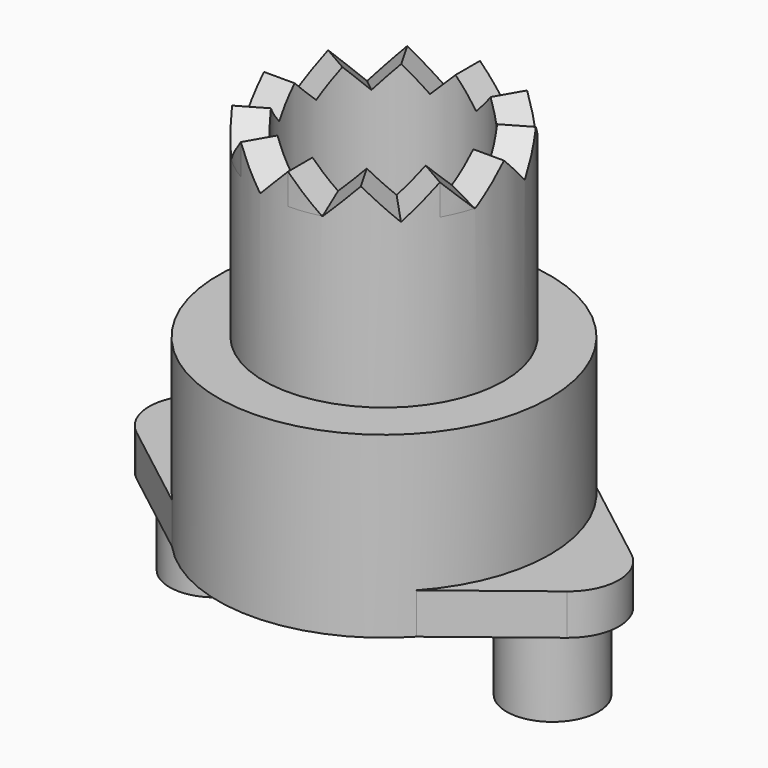
from build123d import *

# Parameters (mm, degrees)
F0_R          = 8.75
F1_DEPTH      = 2
F2_R          = 16.25
F3_DEPTH      = 17.5
F4_R          = 11.75
F5_DEPTH      = 19
F6_R          = 8.75
F7_DEPTH      = 33
F8_R          = 4
F9_DEPTH      = 5.5
F11_DEPTH     = 4
F12_R         = 4.5
F13_DEPTH     = 8
F15_DEPTH     = 22
F17_DEPTH     = 3
F18_SIZE      = 2.99999
F19_SIZE      = 2.99999
F20_DEPTH     = 3
F21_SIZE      = 2.99999
F22_T4_DEPTH  = 18.4300979278
F22_S5_R      = 11.75
F22_T6_DEPTH  = 11
F22_S7_R      = 8.75
F22_T8_DEPTH  = 11
F22_T13_DEPTH = 18.4300979278
F22_S14_R     = 11.75
F22_T15_DEPTH = 12
F22_S17_R     = 8.75
F22_T18_DEPTH = 12
F22_T22_DEPTH = 18.4300979278
F22_S23_R     = 11.75
F22_T24_DEPTH = 12
F22_S25_R     = 8.75
F22_T26_DEPTH = 12
F23_SIZE      = 2.99999
F24_SIZE      = 2.99999
F25_DEPTH     = 3
F26_T4_DEPTH  = 18.4300979278
F26_S5_R      = 11.75
F26_T6_DEPTH  = 12
F26_S7_R      = 8.75
F26_T8_DEPTH  = 12
F26_T12_DEPTH = 18.4300979278
F26_S13_R     = 11.75
F26_T14_DEPTH = 12
F26_S15_R     = 8.75
F26_T16_DEPTH = 12
F26_T20_DEPTH = 18.4300979278
F26_S21_R     = 11.75
F26_T22_DEPTH = 12
F26_S23_R     = 8.75
F26_T24_DEPTH = 12
F26_T28_DEPTH = 18.4300979278
F26_S29_R     = 11.75
F26_T30_DEPTH = 11
F26_S31_R     = 8.75
F26_T32_DEPTH = 11
F26_T36_DEPTH = 18.4300979278
F26_S37_R     = 11.75
F26_T38_DEPTH = 11
F26_S39_R     = 8.75
F26_T40_DEPTH = 11
F26_T44_DEPTH = 18.4300979278
F26_S45_R     = 11.75
F26_T46_DEPTH = 12
F26_S47_R     = 8.75
F26_T48_DEPTH = 12
F26_T52_DEPTH = 18.4300979278
F26_S53_R     = 11.75
F26_T54_DEPTH = 12
F26_S55_R     = 8.75
F26_T56_DEPTH = 12
F26_T60_DEPTH = 18.4300979278
F26_S61_R     = 11.75
F26_T62_DEPTH = 11
F26_S63_R     = 8.75
F26_T64_DEPTH = 11
F26_T68_DEPTH = 18.4300979278
F26_S69_R     = 11.75
F26_T70_DEPTH = 12
F26_S71_R     = 8.75
F26_T72_DEPTH = 12
F26_T76_DEPTH = 18.4300979278
F26_S77_R     = 11.75
F26_T78_DEPTH = 11
F26_S79_R     = 8.75
F26_T80_DEPTH = 11
F26_T84_DEPTH = 18.4300979278
F26_S85_R     = 11.75
F26_T86_DEPTH = 12
F26_S87_R     = 8.75
F26_T88_DEPTH = 12
F26_T92_DEPTH = 18.4300979278
F26_S93_R     = 11.75
F26_T94_DEPTH = 12
F26_S95_R     = 8.75
F26_T96_DEPTH = 12


# Not quite as in the source:
# - a fillet or chamfer that OpenCascade refuses, or shapes differently, is made with other operations: its cross-section is extruded or revolved along the edge and cut away or added
# - a fillet or chamfer is up to 0.001 mm smaller than in the source, because OpenCascade refuses the exact size


with BuildPart() as f1:
    # F0 (on Top) → F1 (new body)
    with BuildSketch(Plane.XY):
        Circle(F0_R)
    extrude(amount=F1_DEPTH)

    # F2 (on face) → F3 (join)
    with BuildSketch(Plane.XY.offset(2)):
        Circle(F2_R)
    extrude(amount=F3_DEPTH)

    # F4 (on face) → F5 (join)
    with BuildSketch(Plane.XY.offset(19.5)):
        Circle(F4_R)
    extrude(amount=F5_DEPTH)

    # F6 (on face) → F7 (cut)
    with BuildSketch(Plane.XY.offset(38.5)):
        Circle(F6_R)
    extrude(amount=-F7_DEPTH, mode=Mode.SUBTRACT)

    # F8 (on face) → F9 (cut, through all)
    with BuildSketch(Plane(origin=(0, 0, 0), x_dir=(1, 0, 0), z_dir=(0, 0, -1))):
        Circle(F8_R)
    extrude(amount=-F9_DEPTH, mode=Mode.SUBTRACT)

    # F10 (on face) → F11 (join)
    with BuildSketch(Plane(origin=(0, 0, 2), x_dir=(1, 0, 0), z_dir=(0, 0, -1))):
        with BuildLine():
            ThreePointArc((-11.9608737139, -11), (-16.25, 0), (-11.9608737139, 11))
            Line((-11.9608737139, 11), (-21.0611990106, 3.9533606738))
            ThreePointArc((-21.0611990106, 3.9533606738), (-23, 0), (-21.0611990106, -3.9533606738))
            Line((-21.0611990106, -3.9533606738), (-11.9608737139, -11))
        make_face()
        with BuildLine():
            Line((21.0611990106, 3.9533606738), (11.9608737139, 11))
            ThreePointArc((11.9608737139, 11), (15.1397935562, 5.9033169553), (16.25, 0))
            ThreePointArc((16.25, 0), (15.1397935562, -5.9033169553), (11.9608737139, -11))
            Line((11.9608737139, -11), (21.0611990106, -3.9533606738))
            ThreePointArc((21.0611990106, -3.9533606738), (23, 0), (21.0611990106, 3.9533606738))
        make_face()
    extrude(amount=-F11_DEPTH)

    # F12 (on face) → F13 (join)
    with BuildSketch(Plane(origin=(0, 0, 2), x_dir=(1, 0, 0), z_dir=(0, 0, -1))):
        with Locations((-16.5, 0)):
            Circle(F12_R)
        with Locations((16.5, 0)):
            Circle(F12_R)
    extrude(amount=F13_DEPTH)

    # F14 (on face) → F15 (join)
    with BuildSketch(Plane.XY.offset(5.5)):
        with BuildLine():
            Line((5.5677643628, -6.75), (-5.5677643628, -6.75))
            ThreePointArc((-5.5677643628, -6.75), (0, -8.75), (5.5677643628, -6.75))
        make_face()
    extrude(amount=F15_DEPTH)

    # F16 (on face) → F17 (cut)
    with BuildSketch(Plane.XY.offset(38.5)):
        with BuildLine():
            ThreePointArc((-7.5777222831, -4.375), (-8.45185098, -2.2646666446), (-8.75, 0))
            Line((-8.75, 0), (-11.75, 0))
            ThreePointArc((-11.75, 0), (-11.3496284589, -3.04112378), (-10.1757984945, -5.875))
            Line((-10.1757984945, -5.875), (-7.5777222831, -4.375))
        make_face()
    extrude(amount=-F17_DEPTH, mode=Mode.SUBTRACT)

    # F18 (size 3 in the source; OpenCascade refuses exactly that, so slightly less here)
    f18_edges = [f1.edges().sort_by_distance(p)[0] for p in [
        (-10.25, 0, 35.5),
    ]]
    chamfer(f18_edges, length=F18_SIZE)

    # F19 (size 3 in the source; OpenCascade refuses exactly that, so slightly less here)
    f19_edges = [f1.edges().sort_by_distance(p)[0] for p in [
        (-8.87676, -5.125, 35.5),
    ]]
    chamfer(f19_edges, length=F19_SIZE)

    # F16 (on face) → F20 (cut)
    with BuildSketch(Plane.XY.offset(38.5)):
        with BuildLine():
            Line((-10.1757984945, 5.875), (-7.5777222831, 4.375))
            ThreePointArc((-7.5777222831, 4.375), (-6.1871843354, 6.1871843354), (-4.375, 7.5777222831))
            Line((-4.375, 7.5777222831), (-5.875, 10.1757984945))
            ThreePointArc((-5.875, 10.1757984945), (-8.3085046789, 8.3085046789), (-10.1757984945, 5.875))
        make_face()
        with BuildLine():
            Line((0, 11.75), (0, 8.75))
            ThreePointArc((0, 8.75), (2.2646666446, 8.45185098), (4.375, 7.5777222831))
            Line((4.375, 7.5777222831), (5.875, 10.1757984945))
            ThreePointArc((5.875, 10.1757984945), (3.04112378, 11.3496284589), (0, 11.75))
        make_face()
        with BuildLine():
            Line((10.1757984945, 5.875), (7.5777222831, 4.375))
            ThreePointArc((7.5777222831, 4.375), (8.45185098, 2.2646666446), (8.75, 0))
            Line((8.75, 0), (11.75, 0))
            ThreePointArc((11.75, 0), (11.3496284589, 3.04112378), (10.1757984945, 5.875))
        make_face()
        with BuildLine():
            ThreePointArc((7.5777222831, -4.375), (6.1871843354, -6.1871843354), (4.375, -7.5777222831))
            Line((4.375, -7.5777222831), (5.875, -10.1757984945))
            ThreePointArc((5.875, -10.1757984945), (8.3085046789, -8.3085046789), (10.1757984945, -5.875))
            Line((10.1757984945, -5.875), (7.5777222831, -4.375))
        make_face()
        with BuildLine():
            ThreePointArc((0, -8.75), (-2.2646666446, -8.45185098), (-4.375, -7.5777222831))
            Line((-4.375, -7.5777222831), (-5.875, -10.1757984945))
            ThreePointArc((-5.875, -10.1757984945), (-3.04112378, -11.3496284589), (0, -11.75))
            Line((0, -11.75), (0, -8.75))
        make_face()
    extrude(amount=-F20_DEPTH, mode=Mode.SUBTRACT)

    # F21 (size 3 in the source; OpenCascade refuses exactly that, so slightly less here)
    f21_edges = [f1.edges().sort_by_distance(p)[0] for p in [
        (5.125, 8.87676, 35.5),
        (8.87676, -5.125, 35.5),
        (0, -10.25, 35.5),
        (-5.125, 8.87676, 35.5),
    ]]
    chamfer(f21_edges, length=F21_SIZE)

    # F22: chamfer of 3 on 3 edges, made by hand


with BuildPart() as f22_tool2:
    # F22_s3 → F22_t4 (new body)
    with BuildSketch(Plane.YZ.offset(1.0349510361)):
        Polygon((3, 35.5), (0, 38.5), (0, 35.5), align=None)
    extrude(amount=F22_T4_DEPTH)

    # F22_s5 → F22_t6 (intersect, symmetric)
    with BuildSketch(Plane.XY.offset(37)):
        Circle(F22_S5_R)
    extrude(amount=F22_T6_DEPTH, both=True, mode=Mode.INTERSECT)

    # F22_s7 → F22_t8 (cut, symmetric)
    with BuildSketch(Plane.XY.offset(37)):
        Circle(F22_S7_R)
    extrude(amount=F22_T8_DEPTH, both=True, mode=Mode.SUBTRACT)

    split(bisect_by=Plane.XY.offset(38.5), keep=Keep.BOTTOM)


with BuildPart() as f1_1:
    add(f1.part)

    # F22_t1: union F22_tool2
    add(f22_tool2.part)


with BuildPart() as f22_tool11:
    # F22_s12 → F22_t13 (new body)
    with BuildSketch(Plane(origin=(0.5174755181, -0.8962938889, 0), x_dir=(0, 0, 1), z_dir=(0.5, -0.8660254038, 0))):
        Polygon((38.5, 0), (35.5, -3), (35.5, 0), align=None)
    extrude(amount=F22_T13_DEPTH)

    # F22_s14 → F22_t15 (intersect, symmetric)
    with BuildSketch(Plane.XY.offset(37)):
        Circle(F22_S14_R)
    extrude(amount=F22_T15_DEPTH, both=True, mode=Mode.INTERSECT)

    split(bisect_by=Plane.XY.offset(38.5), keep=Keep.BOTTOM)

    # F22_s17 → F22_t18 (cut, symmetric)
    with BuildSketch(Plane.XY.offset(37)):
        Circle(F22_S17_R)
    extrude(amount=F22_T18_DEPTH, both=True, mode=Mode.SUBTRACT)


with BuildPart() as f1_2:
    add(f1_1.part)

    # F22_t10: union F22_tool11
    add(f22_tool11.part)


with BuildPart() as f22_tool20:
    # F22_s21 → F22_t22 (new body)
    with BuildSketch(Plane(origin=(-16.8572268886, 9.7325244819, 0), x_dir=(0, 0, 1), z_dir=(0.8660254038, -0.5, 0))):
        Polygon((35.5, -3), (38.5, 0), (35.5, 0), align=None)
    extrude(amount=F22_T22_DEPTH)

    # F22_s23 → F22_t24 (intersect, symmetric)
    with BuildSketch(Plane.XY.offset(37)):
        Circle(F22_S23_R)
    extrude(amount=F22_T24_DEPTH, both=True, mode=Mode.INTERSECT)

    # F22_s25 → F22_t26 (cut, symmetric)
    with BuildSketch(Plane.XY.offset(37)):
        Circle(F22_S25_R)
    extrude(amount=F22_T26_DEPTH, both=True, mode=Mode.SUBTRACT)

    split(bisect_by=Plane.XY.offset(38.5), keep=Keep.BOTTOM)


with BuildPart() as f1_3:
    add(f1_2.part)

    # F22_t19: union F22_tool20
    add(f22_tool20.part)

    # F23 (size 3 in the source; OpenCascade refuses exactly that, so slightly less here)
    f23_edges = [f1_3.edges().sort_by_distance(p)[0] for p in [
        (0, 10.25, 35.5),
        (8.87676, 5.125, 35.5),
    ]]
    chamfer(f23_edges, length=F23_SIZE)

    # F24 (size 3 in the source; OpenCascade refuses exactly that, so slightly less here)
    f24_edges = [f1_3.edges().sort_by_distance(p)[0] for p in [
        (-5.125, -8.87676, 35.5),
    ]]
    chamfer(f24_edges, length=F24_SIZE)

    # F25 (cut): faces of the model
    f25_faces = [f1_3.faces().sort_by_distance(p)[0] for p in [
        (-7.2164850483, -7.2164850483, 38.5),
        (2.6414168537, -9.857901902, 38.5),
        (9.857901902, -2.6414168537, 38.5),
        (7.2164850483, 7.2164850483, 38.5),
        (-2.6414168537, 9.857901902, 38.5),
        (-9.857901902, 2.6414168537, 38.5),
    ]]
    extrude(f25_faces, amount=-F25_DEPTH, mode=Mode.SUBTRACT)

    # F26: chamfer of 3 on 12 edges, made by hand


with BuildPart() as f26_tool2:
    # F26_s3 → F26_t4 (new body)
    with BuildSketch(Plane(origin=(-16.8572268886, 9.7325244819, 0), x_dir=(0, 0, 1), z_dir=(0.8660254038, -0.5, 0))):
        Polygon((35.5, 3), (38.5, 0), (35.5, 0), align=None)
    extrude(amount=F26_T4_DEPTH)

    # F26_s5 → F26_t6 (intersect, symmetric)
    with BuildSketch(Plane.XY.offset(37)):
        Circle(F26_S5_R)
    extrude(amount=F26_T6_DEPTH, both=True, mode=Mode.INTERSECT)

    # F26_s7 → F26_t8 (cut, symmetric)
    with BuildSketch(Plane.XY.offset(37)):
        Circle(F26_S7_R)
    extrude(amount=F26_T8_DEPTH, both=True, mode=Mode.SUBTRACT)


with BuildPart() as f1_4:
    add(f1_3.part)

    # F26_t1: union F26_tool2
    add(f26_tool2.part)


with BuildPart() as f26_tool10:
    # F26_s11 → F26_t12 (new body)
    with BuildSketch(Plane(origin=(-16.8572268886, -9.7325244819, 0), x_dir=(0, 0, 1), z_dir=(0.8660254038, 0.5, 0))):
        Polygon((35.5, 3), (38.5, 0), (35.5, 0), align=None)
    extrude(amount=F26_T12_DEPTH)

    # F26_s13 → F26_t14 (intersect, symmetric)
    with BuildSketch(Plane.XY.offset(37)):
        Circle(F26_S13_R)
    extrude(amount=F26_T14_DEPTH, both=True, mode=Mode.INTERSECT)

    # F26_s15 → F26_t16 (cut, symmetric)
    with BuildSketch(Plane.XY.offset(37)):
        Circle(F26_S15_R)
    extrude(amount=F26_T16_DEPTH, both=True, mode=Mode.SUBTRACT)


with BuildPart() as f1_5:
    add(f1_4.part)

    # F26_t9: union F26_tool10
    add(f26_tool10.part)


with BuildPart() as f26_tool18:
    # F26_s19 → F26_t20 (new body)
    with BuildSketch(Plane(origin=(0.5174755181, -0.8962938889, 0), x_dir=(0, 0, 1), z_dir=(0.5, -0.8660254038, 0))):
        Polygon((38.5, 0), (35.5, 3), (35.5, 0), align=None)
    extrude(amount=F26_T20_DEPTH)

    # F26_s21 → F26_t22 (intersect, symmetric)
    with BuildSketch(Plane.XY.offset(37)):
        Circle(F26_S21_R)
    extrude(amount=F26_T22_DEPTH, both=True, mode=Mode.INTERSECT)

    # F26_s23 → F26_t24 (cut, symmetric)
    with BuildSketch(Plane.XY.offset(37)):
        Circle(F26_S23_R)
    extrude(amount=F26_T24_DEPTH, both=True, mode=Mode.SUBTRACT)


with BuildPart() as f1_6:
    add(f1_5.part)

    # F26_t17: union F26_tool18
    add(f26_tool18.part)


with BuildPart() as f26_tool26:
    # F26_s27 → F26_t28 (new body)
    with BuildSketch(Plane.YZ.offset(1.0349510361)):
        Polygon((0, 38.5), (-3, 35.5), (0, 35.5), align=None)
    extrude(amount=F26_T28_DEPTH)

    # F26_s29 → F26_t30 (intersect, symmetric)
    with BuildSketch(Plane.XY.offset(37)):
        Circle(F26_S29_R)
    extrude(amount=F26_T30_DEPTH, both=True, mode=Mode.INTERSECT)

    # F26_s31 → F26_t32 (cut, symmetric)
    with BuildSketch(Plane.XY.offset(37)):
        Circle(F26_S31_R)
    extrude(amount=F26_T32_DEPTH, both=True, mode=Mode.SUBTRACT)


with BuildPart() as f1_7:
    add(f1_6.part)

    # F26_t25: union F26_tool26
    add(f26_tool26.part)


with BuildPart() as f26_tool34:
    # F26_s35 → F26_t36 (new body)
    with BuildSketch(Plane.XZ.offset(-19.4650489639)):
        Polygon((-3, 35.5), (0, 38.5), (0, 35.5), align=None)
    extrude(amount=F26_T36_DEPTH)

    # F26_s37 → F26_t38 (intersect, symmetric)
    with BuildSketch(Plane.XY.offset(37)):
        Circle(F26_S37_R)
    extrude(amount=F26_T38_DEPTH, both=True, mode=Mode.INTERSECT)

    # F26_s39 → F26_t40 (cut, symmetric)
    with BuildSketch(Plane.XY.offset(37)):
        Circle(F26_S39_R)
    extrude(amount=F26_T40_DEPTH, both=True, mode=Mode.SUBTRACT)


with BuildPart() as f1_8:
    add(f1_7.part)

    # F26_t33: union F26_tool34
    add(f26_tool34.part)


with BuildPart() as f26_tool42:
    # F26_s43 → F26_t44 (new body)
    with BuildSketch(Plane(origin=(16.8572268886, 9.7325244819, 0), x_dir=(0, 0, 1), z_dir=(-0.8660254038, -0.5, 0))):
        Polygon((35.5, 3), (38.5, 0), (35.5, 0), align=None)
    extrude(amount=F26_T44_DEPTH)

    # F26_s45 → F26_t46 (intersect, symmetric)
    with BuildSketch(Plane.XY.offset(37)):
        Circle(F26_S45_R)
    extrude(amount=F26_T46_DEPTH, both=True, mode=Mode.INTERSECT)

    # F26_s47 → F26_t48 (cut, symmetric)
    with BuildSketch(Plane.XY.offset(37)):
        Circle(F26_S47_R)
    extrude(amount=F26_T48_DEPTH, both=True, mode=Mode.SUBTRACT)


with BuildPart() as f1_9:
    add(f1_8.part)

    # F26_t41: union F26_tool42
    add(f26_tool42.part)


with BuildPart() as f26_tool50:
    # F26_s51 → F26_t52 (new body)
    with BuildSketch(Plane(origin=(-0.5174755181, -0.8962938889, 0), x_dir=(0, 0, 1), z_dir=(-0.5, -0.8660254038, 0))):
        Polygon((38.5, 0), (35.5, 3), (35.5, 0), align=None)
    extrude(amount=F26_T52_DEPTH)

    # F26_s53 → F26_t54 (intersect, symmetric)
    with BuildSketch(Plane.XY.offset(37)):
        Circle(F26_S53_R)
    extrude(amount=F26_T54_DEPTH, both=True, mode=Mode.INTERSECT)

    # F26_s55 → F26_t56 (cut, symmetric)
    with BuildSketch(Plane.XY.offset(37)):
        Circle(F26_S55_R)
    extrude(amount=F26_T56_DEPTH, both=True, mode=Mode.SUBTRACT)


with BuildPart() as f1_10:
    add(f1_9.part)

    # F26_t49: union F26_tool50
    add(f26_tool50.part)


with BuildPart() as f26_tool58:
    # F26_s59 → F26_t60 (new body)
    with BuildSketch(Plane.YZ.offset(-1.0349510361)):
        Polygon((0, 38.5), (3, 35.5), (0, 35.5), align=None)
    extrude(amount=-F26_T60_DEPTH)

    # F26_s61 → F26_t62 (intersect, symmetric)
    with BuildSketch(Plane.XY.offset(37)):
        Circle(F26_S61_R)
    extrude(amount=F26_T62_DEPTH, both=True, mode=Mode.INTERSECT)

    # F26_s63 → F26_t64 (cut, symmetric)
    with BuildSketch(Plane.XY.offset(37)):
        Circle(F26_S63_R)
    extrude(amount=F26_T64_DEPTH, both=True, mode=Mode.SUBTRACT)


with BuildPart() as f1_11:
    add(f1_10.part)

    # F26_t57: union F26_tool58
    add(f26_tool58.part)


with BuildPart() as f26_tool66:
    # F26_s67 → F26_t68 (new body)
    with BuildSketch(Plane(origin=(16.8572268886, -9.7325244819, 0), x_dir=(0, 0, 1), z_dir=(-0.8660254038, 0.5, 0))):
        Polygon((35.5, 3), (38.5, 0), (35.5, 0), align=None)
    extrude(amount=F26_T68_DEPTH)

    # F26_s69 → F26_t70 (intersect, symmetric)
    with BuildSketch(Plane.XY.offset(37)):
        Circle(F26_S69_R)
    extrude(amount=F26_T70_DEPTH, both=True, mode=Mode.INTERSECT)

    # F26_s71 → F26_t72 (cut, symmetric)
    with BuildSketch(Plane.XY.offset(37)):
        Circle(F26_S71_R)
    extrude(amount=F26_T72_DEPTH, both=True, mode=Mode.SUBTRACT)


with BuildPart() as f1_12:
    add(f1_11.part)

    # F26_t65: union F26_tool66
    add(f26_tool66.part)


with BuildPart() as f26_tool74:
    # F26_s75 → F26_t76 (new body)
    with BuildSketch(Plane.XZ.offset(19.4650489639)):
        Polygon((3, 35.5), (0, 38.5), (0, 35.5), align=None)
    extrude(amount=-F26_T76_DEPTH)

    # F26_s77 → F26_t78 (intersect, symmetric)
    with BuildSketch(Plane.XY.offset(37)):
        Circle(F26_S77_R)
    extrude(amount=F26_T78_DEPTH, both=True, mode=Mode.INTERSECT)

    # F26_s79 → F26_t80 (cut, symmetric)
    with BuildSketch(Plane.XY.offset(37)):
        Circle(F26_S79_R)
    extrude(amount=F26_T80_DEPTH, both=True, mode=Mode.SUBTRACT)


with BuildPart() as f1_13:
    add(f1_12.part)

    # F26_t73: union F26_tool74
    add(f26_tool74.part)


with BuildPart() as f26_tool82:
    # F26_s83 → F26_t84 (new body)
    with BuildSketch(Plane(origin=(-0.5174755181, 0.8962938889, 0), x_dir=(0, 0, 1), z_dir=(-0.5, 0.8660254038, 0))):
        Polygon((38.5, 0), (35.5, 3), (35.5, 0), align=None)
    extrude(amount=F26_T84_DEPTH)

    # F26_s85 → F26_t86 (intersect, symmetric)
    with BuildSketch(Plane.XY.offset(37)):
        Circle(F26_S85_R)
    extrude(amount=F26_T86_DEPTH, both=True, mode=Mode.INTERSECT)

    # F26_s87 → F26_t88 (cut, symmetric)
    with BuildSketch(Plane.XY.offset(37)):
        Circle(F26_S87_R)
    extrude(amount=F26_T88_DEPTH, both=True, mode=Mode.SUBTRACT)


with BuildPart() as f1_14:
    add(f1_13.part)

    # F26_t81: union F26_tool82
    add(f26_tool82.part)


with BuildPart() as f26_tool90:
    # F26_s91 → F26_t92 (new body)
    with BuildSketch(Plane(origin=(0.5174755181, 0.8962938889, 0), x_dir=(0, 0, 1), z_dir=(0.5, 0.8660254038, 0))):
        Polygon((38.5, 0), (35.5, 3), (35.5, 0), align=None)
    extrude(amount=F26_T92_DEPTH)

    # F26_s93 → F26_t94 (intersect, symmetric)
    with BuildSketch(Plane.XY.offset(37)):
        Circle(F26_S93_R)
    extrude(amount=F26_T94_DEPTH, both=True, mode=Mode.INTERSECT)

    # F26_s95 → F26_t96 (cut, symmetric)
    with BuildSketch(Plane.XY.offset(37)):
        Circle(F26_S95_R)
    extrude(amount=F26_T96_DEPTH, both=True, mode=Mode.SUBTRACT)


with BuildPart() as f1_15:
    add(f1_14.part)

    # F26_t89: union F26_tool90
    add(f26_tool90.part)


solid = f1_15.part
